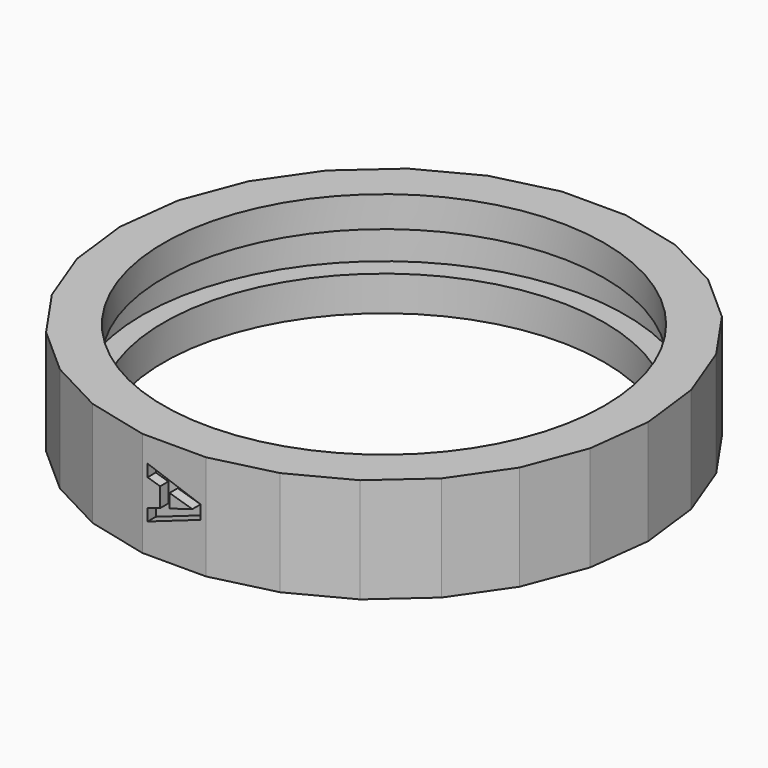
from build123d import *

# Parameters (mm, degrees)
F1_R         = 23
F3_DEPTH     = 10
F1_R_2       = 21
F4_DEPTH     = 3.3333333333
F5_START     = 7.0666666667
F5_DEPTH     = 2.9333333333
F6_TEXT_SIZE = 7.0431932793
F7_DEPTH     = 0.98


# Not quite as in the source:
# - Text() gives the source's letters only with a copy of the font that has no kerning and outlines rounded to 1/6400 em; it was checked with that copy


with BuildPart() as f3:
    # F1 (on Top) → F3 (new body, through all)
    with BuildSketch(Plane.XY):
        Polygon((3.0355495806, 25), (-3.0355495806, 25), (-8.9302336338, 23.5470908713), (-14.3059249684, 20.7257104114), (-18.8502079437, 16.6998269972), (-22.298985351, 11.7034103394), (-24.4518267833, 6.0268340128), (-25.1836169216, 0), (-24.4518267833, -6.0268340128), (-22.298985351, -11.7034103394), (-18.8502079437, -16.6998269972), (-14.3059249684, -20.7257104114), (-8.9302336338, -23.5470908713), (-3.0355495806, -25), (3.0355495806, -25), (8.9302336338, -23.5470908713), (14.3059249684, -20.7257104114), (18.8502079437, -16.6998269972), (22.298985351, -11.7034103394), (24.4518267833, -6.0268340128), (25.1836169216, 0), (24.4518267833, 6.0268340128), (22.298985351, 11.7034103394), (18.8502079437, 16.6998269972), (14.3059249684, 20.7257104114), (8.9302336338, 23.5470908713), align=None)
        Circle(F1_R, mode=Mode.SUBTRACT)
    extrude(amount=F3_DEPTH)

    # F1 (on Top) → F4 (join, through all)
    with BuildSketch(Plane.XY):
        Circle(F1_R)
        Circle(F1_R_2, mode=Mode.SUBTRACT)
    extrude(amount=F4_DEPTH)

    # F1 (on Top) → F5 (join)
    with BuildSketch(Plane.XY.offset(F5_START)):
        Circle(F1_R)
        Circle(F1_R_2, mode=Mode.SUBTRACT)
    extrude(amount=F5_DEPTH)

    # F6 (on face) → F7 (cut)
    with BuildSketch(Plane.XZ.offset(25)):
        with Locations(Location((-2.5355495806, 7.6582552135), (0, 0, -90))):
            Text('A', F6_TEXT_SIZE, font='Open Sans', font_style=FontStyle.BOLD, text_align=(TextAlign.LEFT, TextAlign.BOTTOM))
    extrude(amount=-F7_DEPTH, mode=Mode.SUBTRACT)


solid = f3.part
